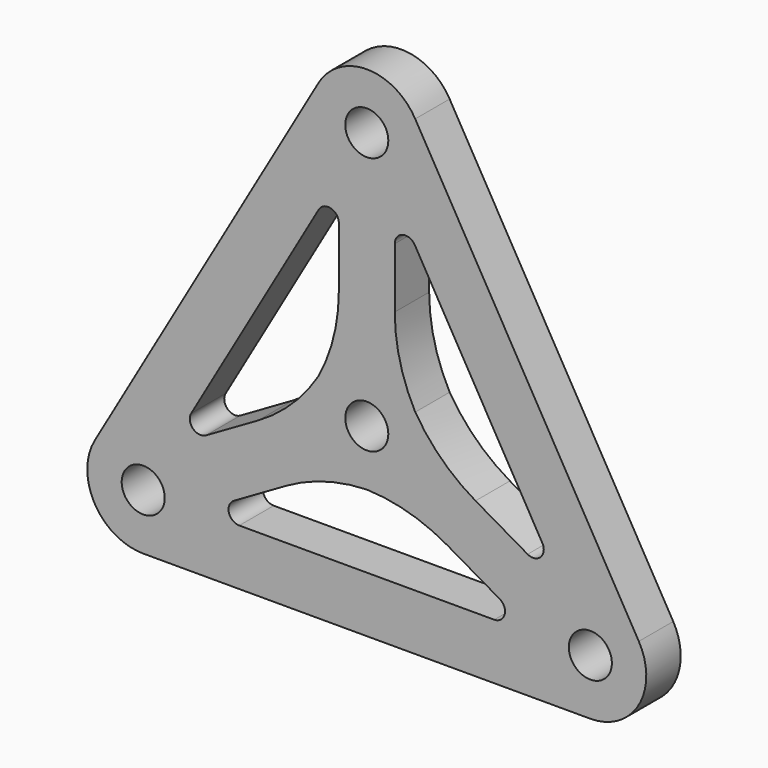
from build123d import *

# Parameters (mm, degrees)
F0_R        = 3.175
F1_DEPTH    = 6.35
F2_R        = 3.175
F3_DEPTH    = 6.351
F5_DEPTH    = 6.351
F6_T1_DEPTH = 6.35
F7_R        = 1.5875


# Not quite as in the source:
# - a fillet or chamfer that OpenCascade refuses, or shapes differently, is made with other operations: its cross-section is extruded or revolved along the edge and cut away or added


with BuildPart() as f1:
    # F0 (on Front) → F1 (new body)
    with BuildSketch(Plane.XZ):
        with BuildLine():
            ThreePointArc((32.9955678842, -27.305), (40.1446075924, -23.1775), (40.1446075924, -14.9225))
            Line((40.1446075924, -14.9225), (7.1490397082, 42.2275))
            ThreePointArc((7.1490397082, 42.2275), (0, 46.355), (-7.1490397082, 42.2275))
            Line((-7.1490397082, 42.2275), (-40.1446075924, -14.9225))
            ThreePointArc((-40.1446075924, -14.9225), (-40.1446075924, -23.1775), (-32.9955678842, -27.305))
            Line((-32.9955678842, -27.305), (32.9955678842, -27.305))
        make_face()
        with Locations((-32.9955678842, -19.05)):
            Circle(F0_R, mode=Mode.SUBTRACT)
        with Locations((32.9955678842, -19.05)):
            Circle(F0_R, mode=Mode.SUBTRACT)
        with Locations((0, 38.1)):
            Circle(F0_R, mode=Mode.SUBTRACT)
    extrude(amount=F1_DEPTH)

    # F2 (on face) → F3 (cut, through all)
    with BuildSketch(Plane.XZ.offset(6.35)):
        Circle(F2_R)
    extrude(amount=-F3_DEPTH, mode=Mode.SUBTRACT)

    # F4 (on face) → F5 (cut, through all)
    with BuildSketch(Plane.XZ.offset(6.35)):
        with BuildLine():
            ThreePointArc((-8.255, 0), (-7.1490397082, 4.1275), (-4.1275, 7.1490397082))
            Line((-4.1275, 7.1490397082), (-4.1275, 30.9509602918))
            Line((-4.1275, 30.9509602918), (-28.8680678842, -11.9009602918))
            Line((-28.8680678842, -11.9009602918), (-8.255, 0))
        make_face()
        with BuildLine():
            Line((24.7405678842, -19.05), (4.1275, -7.1490397082))
            ThreePointArc((4.1275, -7.1490397082), (0, -8.255), (-4.1275, -7.1490397082))
            Line((-4.1275, -7.1490397082), (-24.7405678842, -19.05))
            Line((-24.7405678842, -19.05), (24.7405678842, -19.05))
        make_face()
        with BuildLine():
            ThreePointArc((4.1275, 7.1490397082), (7.1490397082, 4.1275), (8.255, 0))
            Line((8.255, 0), (28.8680678842, -11.9009602918))
            Line((28.8680678842, -11.9009602918), (4.1275, 30.9509602918))
            Line((4.1275, 30.9509602918), (4.1275, 7.1490397082))
        make_face()
    extrude(amount=-F5_DEPTH, mode=Mode.SUBTRACT)

    # F6: fillet of radius 25.4 on 6 edges, made by hand

    # F6_s2 → F6_t1 (join)
    with BuildSketch(Plane.XZ):
        with BuildLine():
            ThreePointArc((-7.2425943396, 3.9610418114), (-4.9185930375, 9.8590537015), (-4.1275, 16.1488627696))
            Line((-4.1275, 16.1488627696), (-4.1275, 7.1490397082))
            ThreePointArc((-4.1275, 7.1490397082), (-5.9042860678, 5.7692660737), (-7.2425943396, 3.9610418114))
        make_face()
        with BuildLine():
            ThreePointArc((-16.0490754007, -4.4999115307), (-10.9974874815, -0.6699003293), (-7.0516600039, 4.2917497817))
            ThreePointArc((-7.0516600039, 4.2917497817), (-7.9484740149, 2.2286286891), (-8.255, 0))
            Line((-8.255, 0), (-16.0490754007, -4.4999115307))
        make_face()
        with BuildLine():
            ThreePointArc((0.1909343357, -8.2527915931), (-6.078894444, -9.1891533721), (-11.9215754007, -11.6489512389))
            Line((-11.9215754007, -11.6489512389), (-4.1275, -7.1490397082))
            ThreePointArc((-4.1275, -7.1490397082), (-2.0441879471, -7.9978947628), (0.1909343357, -8.2527915931))
        make_face()
        with BuildLine():
            ThreePointArc((11.9215754007, -11.6489512389), (6.078894444, -9.1891533721), (-0.1909343357, -8.2527915931))
            ThreePointArc((-0.1909343357, -8.2527915931), (2.0441879471, -7.9978947628), (4.1275, -7.1490397082))
            Line((4.1275, -7.1490397082), (11.9215754007, -11.6489512389))
        make_face()
        with BuildLine():
            ThreePointArc((7.0516600039, 4.2917497817), (10.9974874815, -0.6699003293), (16.0490754007, -4.4999115307))
            Line((16.0490754007, -4.4999115307), (8.255, 0))
            ThreePointArc((8.255, 0), (7.9484740149, 2.2286286891), (7.0516600039, 4.2917497817))
        make_face()
        with BuildLine():
            ThreePointArc((4.1275, 16.1488627696), (4.9185930375, 9.8590537015), (7.2425943396, 3.9610418114))
            ThreePointArc((7.2425943396, 3.9610418114), (5.9042860678, 5.7692660737), (4.1275, 7.1490397082))
            Line((4.1275, 7.1490397082), (4.1275, 16.1488627696))
        make_face()
    extrude(amount=F6_T1_DEPTH)

    # F7
    f7_edges = [f1.edges().sort_by_distance(p)[0] for p in [
        (4.1275, -3.175, 30.95096),
        (-4.1275, -3.175, 30.95096),
        (-28.868068, -3.175, -11.90096),
        (28.868068, -3.175, -11.90096),
        (24.740568, -3.175, -19.05),
        (-24.740568, -3.175, -19.05),
    ]]
    fillet(f7_edges, radius=F7_R)


solid = f1.part
